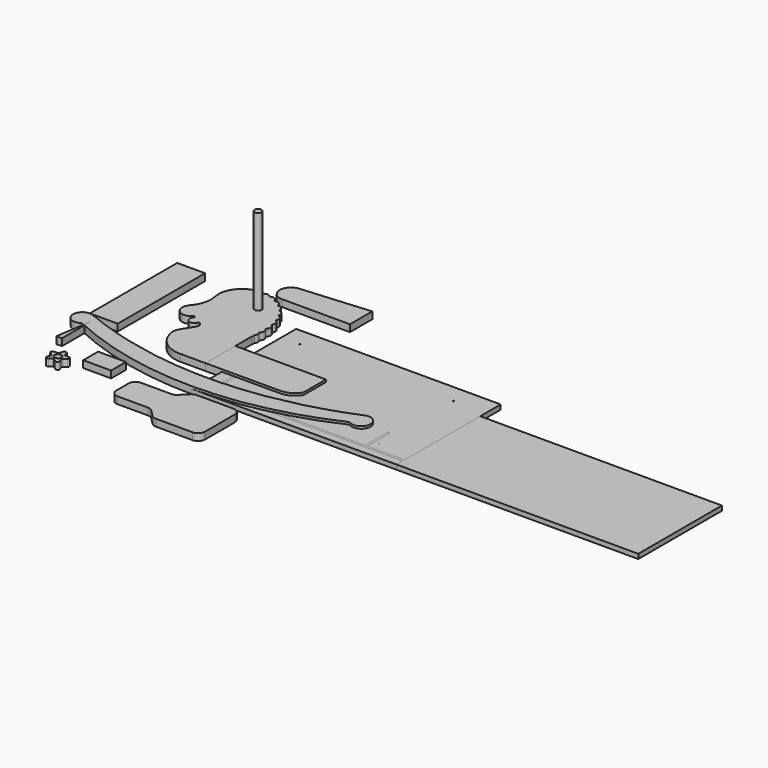
from build123d import *

# Parameters (mm, degrees)
F0_DEPTH     = 19.05
F3_W         = 76.2
F3_H         = 298.45
F6_DEPTH     = 19.05
F7_DEPTH     = 19.05
F8_DEPTH     = 19.05
F24_DEPTH    = 19.05
F9_DEPTH     = 19.05
F1_R         = 9.525
F10_DEPTH    = 19.05
F4_R         = 9.525
F11_DEPTH    = 19.05
F12_W        = 1219.2
F12_H        = 285.75
F13_DEPTH    = 12.7
F14_W        = 76.2
F14_H        = 50.8
F15_DEPTH    = 19.05
F16_W        = 558.8
F16_H        = 355.6
F16_R        = 1.5875
F17_DEPTH    = 12.7
F18_R        = 3.302
F19_DEPTH    = 254
F20_T1_DEPTH = 19.05
F22_DEPTH    = 3.175


# Not quite as in the source:
# - a fillet or chamfer that OpenCascade refuses, or shapes differently, is made with other operations: its cross-section is extruded or revolved along the edge and cut away or added


with BuildPart() as f0:
    # F23 (on Top) → F0 (new body)
    with BuildSketch(Plane.XY):
        with BuildLine():
            ThreePointArc((362.5764395615, 79.7994606567), (365.5156003601, 80.3803434751), (368.3939542349, 79.5489771174))
            ThreePointArc((368.3939542349, 79.5489771174), (406.3507696642, 100.0193427216), (371.2307692308, 125.0461538462))
            ThreePointArc((371.2307692308, 125.0461538462), (305.780467306, 100.5168784657), (238.7266332192, 80.7884546308))
            Line((238.7266332192, 80.7884546308), (151.6675144614, 62.7906814046))
            ThreePointArc((151.6675144614, 62.7906814046), (0, 50.8), (-151.6675144614, 62.7906814046))
            Line((-151.6675144614, 62.7906814046), (-238.7266332192, 80.7884546308))
            ThreePointArc((-238.7266332192, 80.7884546308), (-305.780467306, 100.5168784657), (-371.2307692308, 125.0461538462))
            ThreePointArc((-371.2307692308, 125.0461538462), (-406.3507696642, 100.0193427216), (-368.3939542349, 79.5489771174))
            ThreePointArc((-368.3939542349, 79.5489771174), (-365.5156003601, 80.3803434751), (-362.5764395615, 79.7994606567))
            ThreePointArc((-362.5764395615, 79.7994606567), (0, 0), (362.5764395615, 79.7994606567))
        make_face()
    extrude(amount=F0_DEPTH)

    # F20: fillet of radius 5.08 on 4 edges, made by hand

    # F20_s2 → F20_t1 (join)
    with BuildSketch(Plane.XY):
        with BuildLine():
            ThreePointArc((-238.611869662, 80.7647295058), (-238.7264799862, 80.7898063609), (-238.8404806389, 80.8175232565))
            ThreePointArc((-238.8404806389, 80.8175232565), (-238.7835573714, 80.8029872112), (-238.7266332192, 80.7884546308))
            Line((-238.7266332192, 80.7884546308), (-238.611869662, 80.7647295058))
        make_face()
        with BuildLine():
            ThreePointArc((-151.5514731667, 62.7722250265), (-151.6671191524, 62.7919830902), (-151.7822780186, 62.8144065296))
            Line((-151.7822780186, 62.8144065296), (-151.6675144614, 62.7906814046))
            ThreePointArc((-151.6675144614, 62.7906814046), (-151.6094940949, 62.7814514497), (-151.5514731667, 62.7722250265))
        make_face()
        with BuildLine():
            ThreePointArc((151.7822780186, 62.8144065296), (151.6671191524, 62.7919830902), (151.5514731667, 62.7722250265))
            ThreePointArc((151.5514731667, 62.7722250265), (151.6094940949, 62.7814514497), (151.6675144614, 62.7906814046))
            Line((151.6675144614, 62.7906814046), (151.7822780186, 62.8144065296))
        make_face()
        with BuildLine():
            ThreePointArc((238.8404806389, 80.8175232565), (238.7264799862, 80.7898063609), (238.611869662, 80.7647295058))
            Line((238.611869662, 80.7647295058), (238.7266332192, 80.7884546308))
            ThreePointArc((238.7266332192, 80.7884546308), (238.7835573714, 80.8029872112), (238.8404806389, 80.8175232565))
        make_face()
    extrude(amount=F20_T1_DEPTH)


with BuildPart() as f6:
    # F3 (on Top) → F6 (new body)
    with BuildSketch(Plane.XY):
        with Locations((-342.9, 276.225)):
            Rectangle(F3_W, F3_H)
    extrude(amount=F6_DEPTH)


with BuildPart() as f7:
    # F1 (on Top) → F7 (new body)
    with BuildSketch(Plane.XY):
        with BuildLine():
            Line((-44.45, 203.2), (-165.1, 203.2))
            ThreePointArc((-165.1, 203.2), (-176.8755311223, 198.1592308703), (-185.7009465893, 188.875668598))
            ThreePointArc((-185.7009465893, 188.875668598), (-190.1398197299, 176.8603079346), (-189.4696785207, 164.0687717724))
            Line((-189.4696785207, 164.0687717724), (-188.0272284497, 158.5454996137))
            ThreePointArc((-188.0272284497, 158.5454996137), (-160.8792178475, 117.493976547), (-114.3, 101.6))
            Line((-114.3, 101.6), (-44.45, 101.6))
            Line((-44.45, 101.6), (-44.45, 203.2))
        make_face()
        with BuildLine():
            Line((203.2, 203.2), (-44.45, 203.2))
            Line((-44.45, 203.2), (-44.45, 101.6))
            Line((-44.45, 101.6), (159.2059094878, 101.6))
            ThreePointArc((159.2059094878, 101.6), (183.7855984106, 107.942392187), (202.227727216, 125.3858703758))
            ThreePointArc((202.227727216, 125.3858703758), (202.9520925846, 127.0056601734), (203.2, 128.7626365788))
            Line((203.2, 128.7626365788), (203.2, 203.2))
        make_face()
    extrude(amount=F7_DEPTH)


with BuildPart() as f8:
    # F4 (on Top) → F8 (new body)
    with BuildSketch(Plane.XY):
        Polygon((-355.6, 101.6), (-370.84, 0), (-355.6, 0), align=None)
    extrude(amount=F8_DEPTH)


with BuildPart() as f24:
    # F2 (on Top) → F24 (new body)
    with BuildSketch(Plane.XY):
        with BuildLine():
            Line((-12.3357683632, -55.245), (-95.25, -55.245))
            ThreePointArc((-95.25, -55.245), (-108.7203841816, -60.8246158184), (-114.3, -74.295))
            Line((-114.3, -74.295), (-114.3, -116.205))
            ThreePointArc((-114.3, -116.205), (-108.7203841816, -129.6753841816), (-95.25, -135.255))
            Line((-95.25, -135.255), (-12.3357683632, -135.255))
            ThreePointArc((-12.3357683632, -135.255), (-5.0456489767, -136.7050949057), (1.1346158184, -140.8346158184))
            Line((1.1346158184, -140.8346158184), (19.8203841816, -159.5203841816))
            ThreePointArc((19.8203841816, -159.5203841816), (26.0006489767, -163.6499050943), (33.2907683632, -165.1))
            Line((33.2907683632, -165.1), (133.35, -165.1))
            ThreePointArc((133.35, -165.1), (146.8203841816, -159.5203841816), (152.4, -146.05))
            Line((152.4, -146.05), (152.4, -44.45))
            ThreePointArc((152.4, -44.45), (146.8203841816, -30.9796158184), (133.35, -25.4))
            Line((133.35, -25.4), (33.2907683632, -25.4))
            ThreePointArc((33.2907683632, -25.4), (26.0006489767, -26.8500949057), (19.8203841816, -30.9796158184))
            Line((19.8203841816, -30.9796158184), (1.1346158184, -49.6653841816))
            ThreePointArc((1.1346158184, -49.6653841816), (-5.0456489767, -53.7949050943), (-12.3357683632, -55.245))
        make_face()
    extrude(amount=F24_DEPTH)


with BuildPart() as f9:
    # F5 (on Top) → F9 (new body)
    with BuildSketch(Plane.XY):
        with BuildLine():
            Line((83.8595661674, 434.4131166971), (83.8595661674, 510.6131166971))
            Line((83.8595661674, 510.6131166971), (-104.0407147707, 495.272033835))
            ThreePointArc((-104.0407147707, 495.272033835), (-132.0151526325, 463.6519467574), (-101.5604338326, 434.4131166971))
            Line((-101.5604338326, 434.4131166971), (83.8595661674, 434.4131166971))
        make_face()
    extrude(amount=F9_DEPTH)


with BuildPart() as f10:
    # F1 (on Top) → F10 (new body)
    with BuildSketch(Plane.XY):
        with BuildLine():
            Line((-44.45, 203.2), (-165.1, 203.2))
            ThreePointArc((-165.1, 203.2), (-176.8755311223, 198.1592308703), (-185.7009465893, 188.875668598))
            ThreePointArc((-185.7009465893, 188.875668598), (-190.1398197299, 176.8603079346), (-189.4696785207, 164.0687717724))
            Line((-189.4696785207, 164.0687717724), (-188.0272284497, 158.5454996137))
            ThreePointArc((-188.0272284497, 158.5454996137), (-160.8792178475, 117.493976547), (-114.3, 101.6))
            Line((-114.3, 101.6), (-44.45, 101.6))
            Line((-44.45, 101.6), (-44.45, 203.2))
        make_face()
        with BuildLine():
            ThreePointArc((-185.7009465893, 188.875668598), (-176.8755311223, 198.1592308703), (-165.1, 203.2))
            Line((-165.1, 203.2), (-44.45, 203.2))
            Line((-44.45, 203.2), (-44.45, 259.4098354909))
            ThreePointArc((-44.45, 259.4098354909), (-43.18, 263.6219489746), (-44.45, 267.8340624584))
            ThreePointArc((-44.45, 267.8340624584), (-40.64, 275.7652099163), (-44.45, 283.6963573743))
            ThreePointArc((-44.45, 283.6963573743), (-38.1, 294.6948800024), (-44.45, 305.6934026304))
            ThreePointArc((-44.45, 305.6934026304), (-38.5906947969, 317.5122002176), (-46.3829426599, 328.1562740201))
            ThreePointArc((-46.3829426599, 328.1562740201), (-42.7052552366, 340.8250559769), (-52.2569776763, 349.9238481764))
            ThreePointArc((-52.2569776763, 349.9238481764), (-50.8774453054, 363.0433112557), (-61.8875739433, 370.3097057145))
            ThreePointArc((-61.8875739433, 370.3097057145), (-62.8496748231, 383.4663687774), (-74.9712076133, 388.6713532989))
            ThreePointArc((-74.9712076133, 388.6713532989), (-78.2446195753, 401.4505627885), (-91.095526769, 404.4300938508))
            ThreePointArc((-91.095526769, 404.4300938508), (-96.5770829309, 416.4290922714), (-109.752347363, 417.0892651249))
            ThreePointArc((-109.752347363, 417.0892651249), (-117.2692875993, 427.9298845969), (-130.3536694608, 426.2498928242))
            ThreePointArc((-130.3536694608, 426.2498928242), (-137.1339515676, 432.3115821688), (-146.05, 430.5170394667))
            ThreePointArc((-146.05, 430.5170394667), (-203.789262597, 413.0628732849), (-220.8876864312, 355.2172661506))
            ThreePointArc((-220.8876864312, 355.2172661506), (-221.7624895657, 320.1230915048), (-238.2774433701, 289.1453143827))
            ThreePointArc((-238.2774433701, 289.1453143827), (-236.4411807463, 253.6847983691), (-200.9479518855, 254.709864909))
            ThreePointArc((-200.9479518855, 254.709864909), (-196.2789288711, 254.7913025598), (-196.1974912203, 250.1222795454))
            ThreePointArc((-196.1974912203, 250.1222795454), (-193.664280563, 230.4510480441), (-175.0285663074, 237.2396163169))
            ThreePointArc((-175.0285663074, 237.2396163169), (-173.1117688621, 239.2554829488), (-170.3349104142, 239.0915076939))
            ThreePointArc((-170.3349104142, 239.0915076939), (-164.0809192618, 231.1736229522), (-165.573630811, 221.1947895359))
            Line((-165.573630811, 221.1947895359), (-185.7009465893, 188.875668598))
        make_face()
        with Locations((-114.3, 368.3)):
            Circle(F1_R, mode=Mode.SUBTRACT)
    extrude(amount=F10_DEPTH)

    # F18
    f18_edges = [f10.edges().sort_by_distance(p)[0] for p in [
        (-146.05, 430.517039, 9.525),
        (-130.353669, 426.249893, 9.525),
        (-109.752347, 417.089265, 9.525),
        (-91.095527, 404.430094, 9.525),
        (-74.971208, 388.671353, 9.525),
        (-61.887574, 370.309706, 9.525),
        (-52.256978, 349.923848, 9.525),
        (-46.382943, 328.156274, 9.525),
        (-44.45, 305.693403, 9.525),
        (-44.45, 283.696357, 9.525),
        (-44.45, 267.834062, 9.525),
        (-44.45, 259.409835, 9.525),
    ]]
    fillet(f18_edges, radius=F18_R)


with BuildPart() as f11:
    # F4 (on Top) → F11 (new body)
    with BuildSketch(Plane.XY):
        with BuildLine():
            Line((-320.878053669, -58.3774367637), (-330.3112728965, -58.3774367637))
            ThreePointArc((-330.3112728965, -58.3774367637), (-335.1426399993, -61.8876304323), (-333.2972219781, -67.5672430952))
            Line((-333.2972219781, -67.5672430952), (-325.6655873114, -73.1119502387))
            ThreePointArc((-325.6655873114, -73.1119502387), (-324.4660655977, -74.7629502387), (-324.4660655977, -76.8036984696))
            Line((-324.4660655977, -76.8036984696), (-327.3810906507, -85.7752230855))
            ThreePointArc((-327.3810906507, -85.7752230855), (-325.5356726295, -91.4548357483), (-319.5637744662, -91.4548357483))
            Line((-319.5637744662, -91.4548357483), (-311.9321397995, -85.9101286048))
            ThreePointArc((-311.9321397995, -85.9101286048), (-309.9912728965, -85.2795027202), (-308.0504059934, -85.9101286048))
            Line((-308.0504059934, -85.9101286048), (-300.4187713267, -91.4548357483))
            ThreePointArc((-300.4187713267, -91.4548357483), (-294.4468731634, -91.4548357483), (-292.6014551423, -85.7752230855))
            Line((-292.6014551423, -85.7752230855), (-295.5164801953, -76.8036984696))
            ThreePointArc((-295.5164801953, -76.8036984696), (-295.5164801953, -74.7629502387), (-294.3169584815, -73.1119502387))
            Line((-294.3169584815, -73.1119502387), (-286.6853238148, -67.5672430952))
            ThreePointArc((-286.6853238148, -67.5672430952), (-284.8399057937, -61.8876304323), (-289.6712728965, -58.3774367637))
            Line((-289.6712728965, -58.3774367637), (-299.1044921239, -58.3774367637))
            ThreePointArc((-299.1044921239, -58.3774367637), (-301.045359027, -57.7468108792), (-302.2448807407, -56.0958108792))
            Line((-302.2448807407, -56.0958108792), (-305.1599057937, -47.1242862632))
            ThreePointArc((-305.1599057937, -47.1242862632), (-309.9912728965, -43.6140925947), (-314.8226399993, -47.1242862632))
            Line((-314.8226399993, -47.1242862632), (-317.7376650522, -56.0958108792))
            ThreePointArc((-317.7376650522, -56.0958108792), (-318.9371867659, -57.7468108792), (-320.878053669, -58.3774367637))
        make_face()
        with Locations((-309.9912728965, -70.0598049912)):
            Circle(F4_R, mode=Mode.SUBTRACT)
    extrude(amount=F11_DEPTH)


with BuildPart() as f13:
    # F12 (on Top) → F13 (new body)
    with BuildSketch(Plane.XY):
        with Locations((609.6, 142.875)):
            Rectangle(F12_W, F12_H)
    extrude(amount=F13_DEPTH)


with BuildPart() as f15:
    # F14 (on Top) → F15 (new body)
    with BuildSketch(Plane.XY):
        with Locations((-218.6286854506, -25.4)):
            Rectangle(F14_W, F14_H)
    extrude(amount=F15_DEPTH)


with BuildPart() as f17:
    # F16 (on Top) → F17 (new body)
    with BuildSketch(Plane.XY):
        with Locations((279.4, 177.8)):
            Rectangle(F16_W, F16_H)
        with Locations((50.8, 25.4)):
            Circle(F16_R, mode=Mode.SUBTRACT)
        with Locations((36.5125, 50.8)):
            Circle(F16_R, mode=Mode.SUBTRACT)
        with Locations((50.8, 50.8)):
            Circle(F16_R, mode=Mode.SUBTRACT)
        with Locations((469.9, 25.4)):
            Circle(F16_R, mode=Mode.SUBTRACT)
        with Locations((469.9, 50.8)):
            Circle(F16_R, mode=Mode.SUBTRACT)
        with Locations((50.8, 304.8)):
            Circle(F16_R, mode=Mode.SUBTRACT)
        with Locations((469.9, 304.8)):
            Circle(F16_R, mode=Mode.SUBTRACT)
    extrude(amount=F17_DEPTH)

    # F21 (on face) → F22 (cut)
    with BuildSketch(Plane.XY.offset(12.7)):
        with BuildLine():
            Line((558.8, 20.6375), (558.8, 26.9875))
            Line((558.8, 26.9875), (457.2, 26.9875))
            Line((457.2, 26.9875), (457.2, 103.1875))
            ThreePointArc((457.2, 103.1875), (454.025, 100.0125), (450.85, 103.1875))
            Line((450.85, 103.1875), (450.85, 26.9875))
            Line((450.85, 26.9875), (38.1, 26.9875))
            Line((38.1, 26.9875), (38.1, 103.1875))
            ThreePointArc((38.1, 103.1875), (34.925, 106.3625), (31.75, 103.1875))
            Line((31.75, 103.1875), (31.75, 26.9875))
            Line((31.75, 26.9875), (19.05, 26.9875))
            ThreePointArc((19.05, 26.9875), (15.875, 23.8125), (19.05, 20.6375))
            Line((19.05, 20.6375), (558.8, 20.6375))
        make_face()
        with BuildLine():
            ThreePointArc((450.85, 103.1875), (454.025, 100.0125), (457.2, 103.1875))
            ThreePointArc((457.2, 103.1875), (454.025, 106.3625), (450.85, 103.1875))
        make_face()
    extrude(amount=-F22_DEPTH, mode=Mode.SUBTRACT)


with BuildPart() as f19:
    # F1 (on Top) → F19 (new body)
    with BuildSketch(Plane.XY):
        with Locations((-114.3, 368.3)):
            Circle(F1_R)
    extrude(amount=F19_DEPTH)


solid = Compound([f0.part, f6.part, f7.part, f8.part, f24.part, f9.part, f10.part, f11.part, f13.part, f15.part, f17.part, f19.part])
